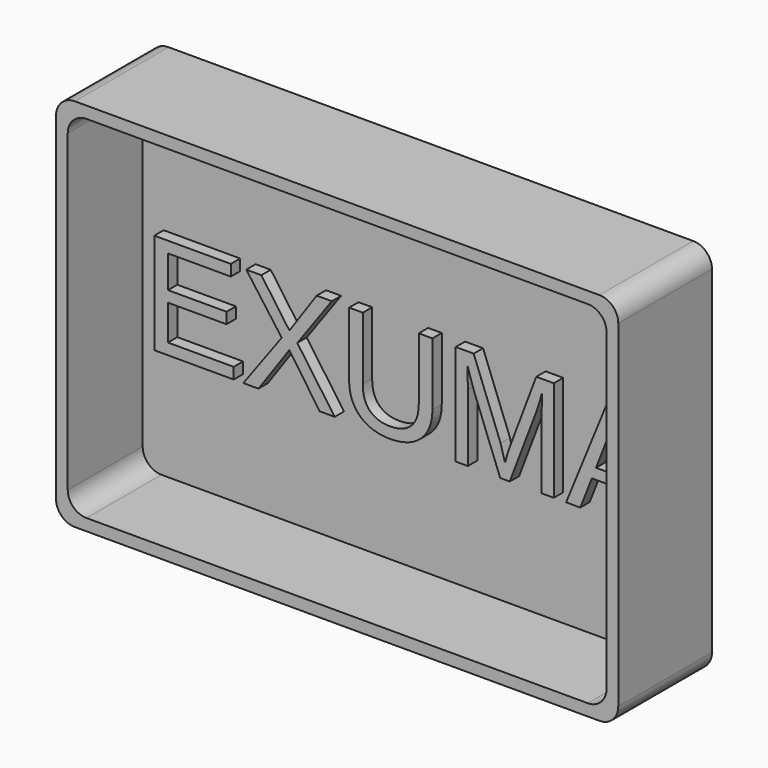
from build123d import *

# Parameters (mm, degrees)
F0_W         = 152.4
F0_H         = 101.6
F1_DEPTH     = 6.35
F2_W         = 152.4
F2_H         = 101.6
F2_W_2       = 146.05
F2_H_2       = 95.25
F3_DEPTH     = 25.4
F4_R         = 5.08
F5_TEXT_SIZE = 39.7398641023
F6_DEPTH     = 3.175


# Not quite as in the source:
# - Text() gives the source's letters only with a copy of the font that has no kerning and outlines rounded to 1/6400 em; it was checked with that copy


with BuildPart() as f1:
    # F0 (on Front) → F1 (new body)
    with BuildSketch(Plane.XZ):
        with Locations((6.1326734722, 1.857150434)):
            Rectangle(F0_W, F0_H)
    extrude(amount=F1_DEPTH)

    # F2 (on face) → F3 (join)
    with BuildSketch(Plane.XZ.offset(6.35)):
        with Locations((6.1326734722, 1.857150434)):
            Rectangle(F2_W, F2_H)
        with Locations((6.1326734722, 1.857150434)):
            Rectangle(F2_W_2, F2_H_2, mode=Mode.SUBTRACT)
    extrude(amount=F3_DEPTH)

    # F4
    f4_edges = [f1.edges().sort_by_distance(p)[0] for p in [
        (-70.067327, -15.875, -48.94285),
        (-66.892327, -19.05, -45.76785),
        (-66.892327, -19.05, 49.48215),
        (-70.067327, -15.875, 52.65715),
        (82.332673, -15.875, -48.94285),
        (79.157673, -19.05, -45.76785),
        (82.332673, -15.875, 52.65715),
        (79.157673, -19.05, 49.48215),
    ]]
    fillet(f4_edges, radius=F4_R)

    # F5 (on face) → F6 (join)
    with BuildSketch(Plane.XZ.offset(6.35)):
        with Locations((-64.4804351032, -14.5596088842)):
            Text('EXUMA', F5_TEXT_SIZE, font='Arimo', text_align=(TextAlign.LEFT, TextAlign.BOTTOM))
    extrude(amount=F6_DEPTH)


solid = f1.part
